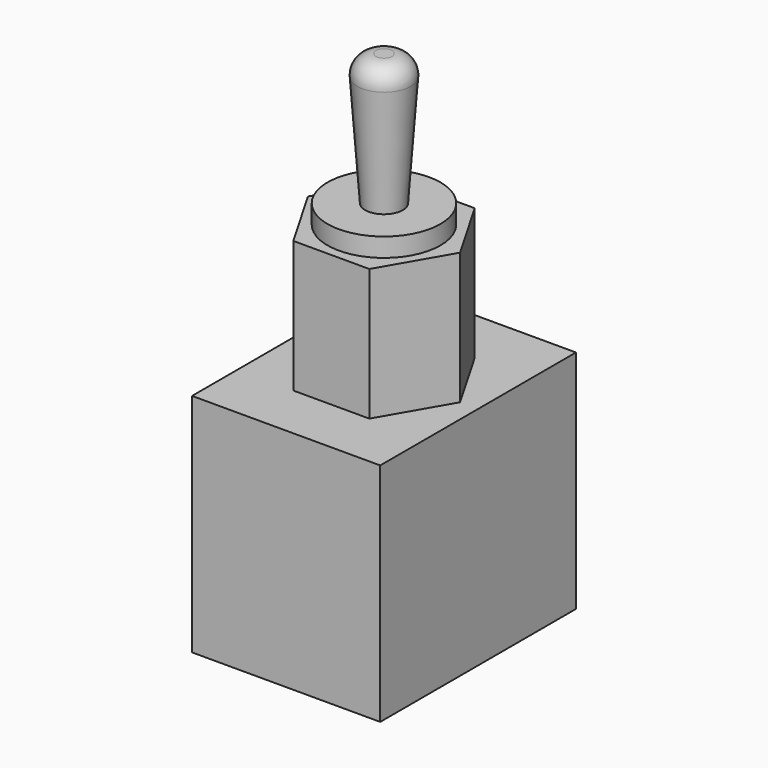
from build123d import *

# Parameters (mm, degrees)
F0_W     = 10
F0_H     = 13
F1_DEPTH = 12
F2_DEPTH = 7
F3_R     = 3
F4_DEPTH = 1
F5_R     = 1
F7_R     = 1.5
F9_R     = 1


with BuildPart() as f1:
    # F0 (on Top) → F1 (new body)
    with BuildSketch(Plane.XY):
        Rectangle(F0_W, F0_H)
        Polygon((4.0414518843, 0), (2.0207259422, -3.5), (-2.0207259422, -3.5), (-4.0414518843, 0), (-2.0207259422, 3.5), (2.0207259422, 3.5), align=None, mode=Mode.SUBTRACT)
        Polygon((-2.0207259422, -3.5), (2.0207259422, -3.5), (4.0414518843, 0), (2.0207259422, 3.5), (-2.0207259422, 3.5), (-4.0414518843, 0), align=None)
    extrude(amount=-F1_DEPTH)

    # F0 (on Top) → F2 (join)
    with BuildSketch(Plane.XY):
        Polygon((-2.0207259422, -3.5), (2.0207259422, -3.5), (4.0414518843, 0), (2.0207259422, 3.5), (-2.0207259422, 3.5), (-4.0414518843, 0), align=None)
    extrude(amount=F2_DEPTH)

    # F3 (on face) → F4 (join)
    with BuildSketch(Plane.XY.offset(7)):
        Circle(F3_R)
    extrude(amount=F4_DEPTH)


with BuildPart() as f8:
    # F5 (on face) → F8 section 0
    with BuildSketch(Plane.XY.offset(8)):
        Circle(F5_R)
    # F7 (on offset) → F8 section 1
    with BuildSketch(Plane.XY.offset(15)):
        Circle(F7_R)
    loft()

    # F9
    f9_edges = [f8.edges().sort_by_distance(p)[0] for p in [
        (-1.5, 0, 15),
    ]]
    fillet(f9_edges, radius=F9_R)


solid = Compound([f1.part, f8.part])
